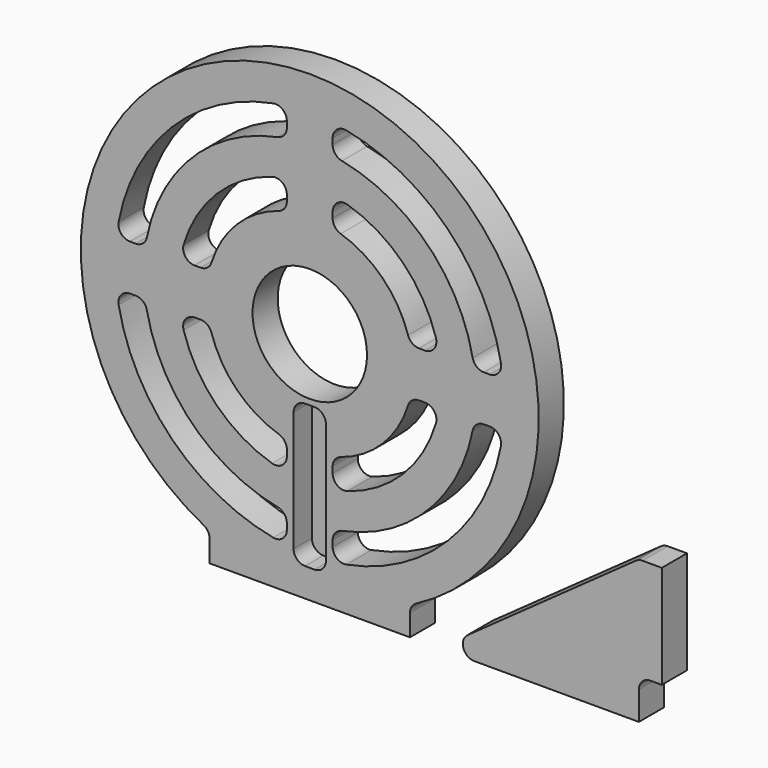
from build123d import *

# Parameters (mm, degrees)
F0_R      = 40
F0_R_2    = 10
F1_DEPTH  = 2.75
F3_DEPTH  = 5.5
F5_DEPTH  = 5.5
F6_R      = 2
F6_2_R    = 2
F7_W      = 4
F7_H      = 18
F8_DEPTH  = 5.5
F9_R      = 2
F10_W     = 5.65
F10_H     = 25
F11_DEPTH = 4
F12_R     = 2


with BuildPart() as f1:
    # F0 (on Front) → F1 (new body, symmetric)
    with BuildSketch(Plane.XZ):
        Circle(F0_R)
        with BuildLine():
            ThreePointArc((-4, -33.7638860323), (-24.0416305603, -24.0416305603), (-33.7638860323, -4))
            Line((-33.7638860323, -4), (-28.7228132327, -4))
            ThreePointArc((-28.7228132327, -4), (-20.5060966544, -20.5060966544), (-4, -28.7228132327))
            Line((-4, -28.7228132327), (-4, -33.7638860323))
        make_face(mode=Mode.SUBTRACT)
        with BuildLine():
            ThreePointArc((-17.5499287748, -4), (-12.7279220614, -12.7279220614), (-4, -17.5499287748))
            Line((-4, -17.5499287748), (-4, -22.6495033058))
            ThreePointArc((-4, -22.6495033058), (-16.2634559673, -16.2634559673), (-22.6495033058, -4))
            Line((-22.6495033058, -4), (-17.5499287748, -4))
        make_face(mode=Mode.SUBTRACT)
        with BuildLine():
            ThreePointArc((4, -28.7228132327), (20.5060966544, -20.5060966544), (28.7228132327, -4))
            Line((28.7228132327, -4), (33.7638860323, -4))
            ThreePointArc((33.7638860323, -4), (24.0416305603, -24.0416305603), (4, -33.7638860323))
            Line((4, -33.7638860323), (4, -28.7228132327))
        make_face(mode=Mode.SUBTRACT)
        with BuildLine():
            Line((4, -22.6495033058), (4, -17.5499287748))
            ThreePointArc((4, -17.5499287748), (12.7279220614, -12.7279220614), (17.5499287748, -4))
            Line((17.5499287748, -4), (22.6495033058, -4))
            ThreePointArc((22.6495033058, -4), (16.2634559673, -16.2634559673), (4, -22.6495033058))
        make_face(mode=Mode.SUBTRACT)
        with BuildLine():
            Line((-4, 22.6495033058), (-4, 17.5499287748))
            ThreePointArc((-4, 17.5499287748), (-12.7279220614, 12.7279220614), (-17.5499287748, 4))
            Line((-17.5499287748, 4), (-22.6495033058, 4))
            ThreePointArc((-22.6495033058, 4), (-16.2634559673, 16.2634559673), (-4, 22.6495033058))
        make_face(mode=Mode.SUBTRACT)
        with BuildLine():
            ThreePointArc((-33.7638860323, 4), (-24.0416305603, 24.0416305603), (-4, 33.7638860323))
            Line((-4, 33.7638860323), (-4, 28.7228132327))
            ThreePointArc((-4, 28.7228132327), (-20.5060966544, 20.5060966544), (-28.7228132327, 4))
            Line((-28.7228132327, 4), (-33.7638860323, 4))
        make_face(mode=Mode.SUBTRACT)
        Circle(F0_R_2, mode=Mode.SUBTRACT)
        with BuildLine():
            Line((22.6495033058, 4), (17.5499287748, 4))
            ThreePointArc((17.5499287748, 4), (12.7279220614, 12.7279220614), (4, 17.5499287748))
            Line((4, 17.5499287748), (4, 22.6495033058))
            ThreePointArc((4, 22.6495033058), (16.2634559673, 16.2634559673), (22.6495033058, 4))
        make_face(mode=Mode.SUBTRACT)
        with BuildLine():
            ThreePointArc((28.7228132327, 4), (20.5060966544, 20.5060966544), (4, 28.7228132327))
            Line((4, 28.7228132327), (4, 33.7638860323))
            ThreePointArc((4, 33.7638860323), (24.0416305603, 24.0416305603), (33.7638860323, 4))
            Line((33.7638860323, 4), (28.7228132327, 4))
        make_face(mode=Mode.SUBTRACT)
    extrude(amount=F1_DEPTH, both=True)

    # F2 (on face) → F3 (join)
    with BuildSketch(Plane.XZ.offset(2.75)):
        with BuildLine():
            ThreePointArc((17.5, -35.9687364248), (0, -40), (-17.5, -35.9687364248))
            Line((-17.5, -35.9687364248), (-17.5, -40.9687364248))
            Line((-17.5, -40.9687364248), (17.5, -40.9687364248))
            Line((17.5, -40.9687364248), (17.5, -35.9687364248))
        make_face()
    extrude(amount=-F3_DEPTH)

    # F6
    f6_edges = [f1.edges().sort_by_distance(p)[0] for p in [
        (17.549929, 0, 4),
        (28.722813, 0, 4),
        (4, 0, 28.722813),
        (-22.649503, 0, 4),
        (-4, 0, 28.722813),
        (-28.722813, 0, 4),
        (-17.549929, 0, 4),
        (-4, 0, 17.549929),
        (4, 0, 33.763886),
        (33.763886, 0, 4),
        (-4, 0, 33.763886),
        (-33.763886, 0, 4),
        (-17.549929, 0, -4),
        (-28.722813, 0, -4),
        (28.722813, 0, -4),
        (4, 0, -28.722813),
        (33.763886, 0, -4),
        (22.649503, 0, -4),
        (-4, 0, -28.722813),
        (-33.763886, 0, -4),
        (-22.649503, 0, -4),
        (-4, 0, -33.763886),
        (4, 0, -33.763886),
        (22.649503, 0, 4),
        (-4, 0, 22.649503),
        (-4, 0, -17.549929),
        (4, 0, -22.649503),
        (-4, 0, -22.649503),
        (-17.5, 0, -35.968736),
        (17.5, 0, -35.968736),
        (4, 0, 22.649503),
        (4, 0, 17.549929),
        (17.549929, 0, -4),
        (4, 0, -17.549929),
    ]]
    fillet(f6_edges, radius=F6_R)

    # F10 (on face) → F11 (cut)
    with BuildSketch(Plane.XZ.offset(2.75)):
        with Locations((0, -23.4687364248)):
            Rectangle(F10_W, F10_H)
    extrude(amount=-F11_DEPTH, mode=Mode.SUBTRACT)

    # F12
    f12_edges = [f1.edges().sort_by_distance(p)[0] for p in [
        (-2.825, -0.75, -10.968736),
        (2.825, -0.75, -10.968736),
        (2.825, -0.75, -35.968736),
        (-2.825, -0.75, -35.968736),
    ]]
    fillet(f12_edges, radius=F12_R)


with BuildPart() as f5:
    # F4 (on face) → F5 (new body)
    with BuildSketch(Plane.XZ.offset(2.75)):
        Polygon((57.5, -15.9687364248), (22.5, -40.9687364248), (57.5, -40.9687364248), align=None)
    extrude(amount=-F5_DEPTH)

    # F6#2
    f6_2_edges = [f5.edges().sort_by_distance(p)[0] for p in [
        (22.5, 0, -40.968736),
    ]]
    fillet(f6_2_edges, radius=F6_2_R)

    # F7 (on face) → F8 (join)
    with BuildSketch(Plane.XZ.offset(2.75)):
        with Locations((59.5, -24.9687364248)):
            Rectangle(F7_W, F7_H)
    extrude(amount=-F8_DEPTH)

    # F9
    f9_edges = [f5.edges().sort_by_distance(p)[0] for p in [
        (57.5, 0, -33.968736),
        (57.5, 0, -15.968736),
    ]]
    fillet(f9_edges, radius=F9_R)


solid = Compound([f1.part, f5.part])
